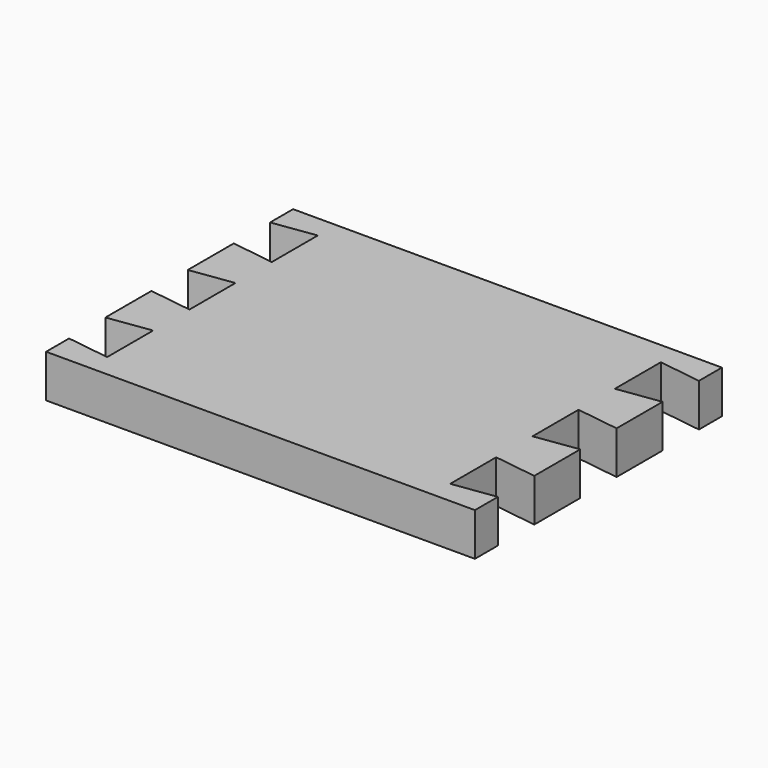
from build123d import *

# Parameters (mm, degrees)
F0_W     = 635
F0_H     = 457.2
F1_DEPTH = 63.5
F3_DEPTH = 63.501


# Not quite as in the source:
# - a pattern or mirror of a feature is missing from the dataset's text; its kind, count and spacing are read off the source's solid


with BuildPart() as f1:
    # F0 (on Top) → F1 (new body)
    with BuildSketch(Plane.XY):
        with Locations((317.5, -228.6)):
            Rectangle(F0_W, F0_H)
    extrude(amount=-F1_DEPTH)

    # F2 (on Top) → F3 (cut, through all)
    with BuildSketch(Plane.XY):
        Polygon((63.5, -33.6378284982), (0, -42.5621715018), (0, -109.8378284982), (63.5, -118.7621715018), align=None)
        Polygon((63.5, -186.0378284982), (0, -194.9621715018), (0, -262.2378284982), (63.5, -271.1621715018), align=None)
        Polygon((63.5, -338.4378284982), (0, -347.3621715018), (0, -414.6378284982), (63.5, -423.5621715018), align=None)
    f3 = extrude(amount=-F3_DEPTH, mode=Mode.SUBTRACT)

    # F3_copies: F3 across plane
    add(f3.mirror(Plane(origin=(317.5, 0, 0), x_dir=(0, 0, 1), z_dir=(1, 0, 0))), mode=Mode.SUBTRACT)


solid = f1.part
